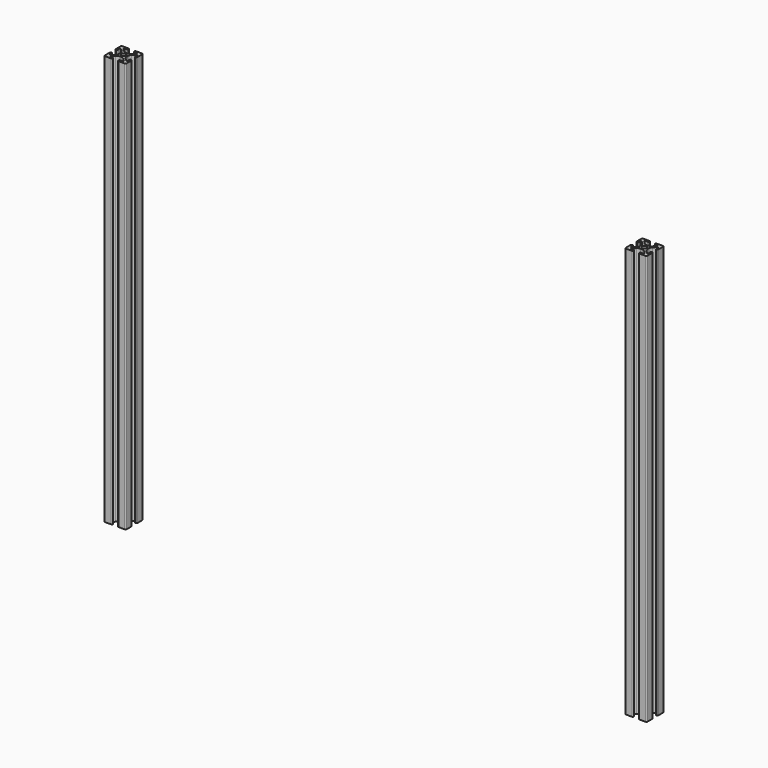
from build123d import *

# Parameters (mm, degrees)
F0_R     = 2.6035
F1_DEPTH = 480.06
F2_R     = 1.18109
F3_R     = 5.08
F4_R     = 0.762
F5_R     = 1.27


# Not quite as in the source:
# - a fillet or chamfer is up to 0.001 mm smaller than in the source, because OpenCascade refuses the exact size


with BuildPart() as f1:
    # F0 (on Top) → F1 (new body)
    with BuildSketch(Plane.XY):
        Polygon((12.7, 3.2385), (12.7, 12.7), (3.2385, 12.7), (3.2385, 10.3378), (8.7752354349, 10.3378), (2.9459354349, 4.5085), (-2.9459354349, 4.5085), (-8.7752354349, 10.3378), (-3.2385, 10.3378), (-3.2385, 12.7), (-12.7, 12.7), (-12.7, 3.2385), (-10.3378, 3.2385), (-10.3378, 8.7752354349), (-4.5085, 2.9459354349), (-4.5085, -2.9459354349), (-10.3378, -8.7752354349), (-10.3378, -3.2385), (-12.7, -3.2385), (-12.7, -12.7), (-3.2385, -12.7), (-3.2385, -10.3378), (-8.7752354349, -10.3378), (-2.9459354349, -4.5085), (2.9459354349, -4.5085), (8.7752354349, -10.3378), (3.2385, -10.3378), (3.2385, -12.7), (12.7, -12.7), (12.7, -3.2385), (10.3378, -3.2385), (10.3378, -8.7752354349), (4.5085, -2.9459354349), (4.5085, 2.9459354349), (10.3378, 8.7752354349), (10.3378, 3.2385), align=None)
        Circle(F0_R, mode=Mode.SUBTRACT)
    extrude(amount=F1_DEPTH)

    # F2 (radius 1.1811 in the source; OpenCascade refuses exactly that, so slightly less here)
    f2_edges = [f1.edges().sort_by_distance(p)[0] for p in [
        (3.2385, 12.7, 240.03),
        (3.2385, 10.3378, 240.03),
        (-3.2385, 12.7, 240.03),
        (-12.7, 3.2385, 240.03),
        (-3.2385, 10.3378, 240.03),
        (-10.3378, 3.2385, 240.03),
        (12.7, 3.2385, 240.03),
        (10.3378, 3.2385, 240.03),
        (12.7, -3.2385, 240.03),
        (10.3378, -3.2385, 240.03),
        (3.2385, -10.3378, 240.03),
        (-3.2385, -10.3378, 240.03),
        (-10.3378, -3.2385, 240.03),
        (-12.7, -3.2385, 240.03),
        (-3.2385, -12.7, 240.03),
        (3.2385, -12.7, 240.03),
    ]]
    fillet(f2_edges, radius=F2_R)

    # F3
    f3_edges = [f1.edges().sort_by_distance(p)[0] for p in [
        (2.945935, 4.5085, 240.03),
        (-2.945935, 4.5085, 240.03),
        (4.5085, -2.945935, 240.03),
        (4.5085, 2.945935, 240.03),
        (2.945935, -4.5085, 240.03),
        (-2.945935, -4.5085, 240.03),
        (-4.5085, -2.945935, 240.03),
        (-4.5085, 2.945935, 240.03),
    ]]
    fillet(f3_edges, radius=F3_R)

    # F4
    f4_edges = [f1.edges().sort_by_distance(p)[0] for p in [
        (8.775235, 10.3378, 240.03),
        (-8.775235, 10.3378, 240.03),
        (-10.3378, 8.775235, 240.03),
        (-10.3378, -8.775235, 240.03),
        (-8.775235, -10.3378, 240.03),
        (8.775235, -10.3378, 240.03),
        (10.3378, -8.775235, 240.03),
        (10.3378, 8.775235, 240.03),
    ]]
    fillet(f4_edges, radius=F4_R)

    # F5
    f5_edges = [f1.edges().sort_by_distance(p)[0] for p in [
        (-12.7, -12.7, 240.03),
        (12.7, -12.7, 240.03),
        (12.7, 12.7, 240.03),
        (-12.7, 12.7, 240.03),
    ]]
    fillet(f5_edges, radius=F5_R)


with BuildPart() as f6_1:
    # F6: copy of F1
    add(f1.part.moved(Location((609.6, 0, 0))))


solid = Compound([f1.part, f6_1.part])
